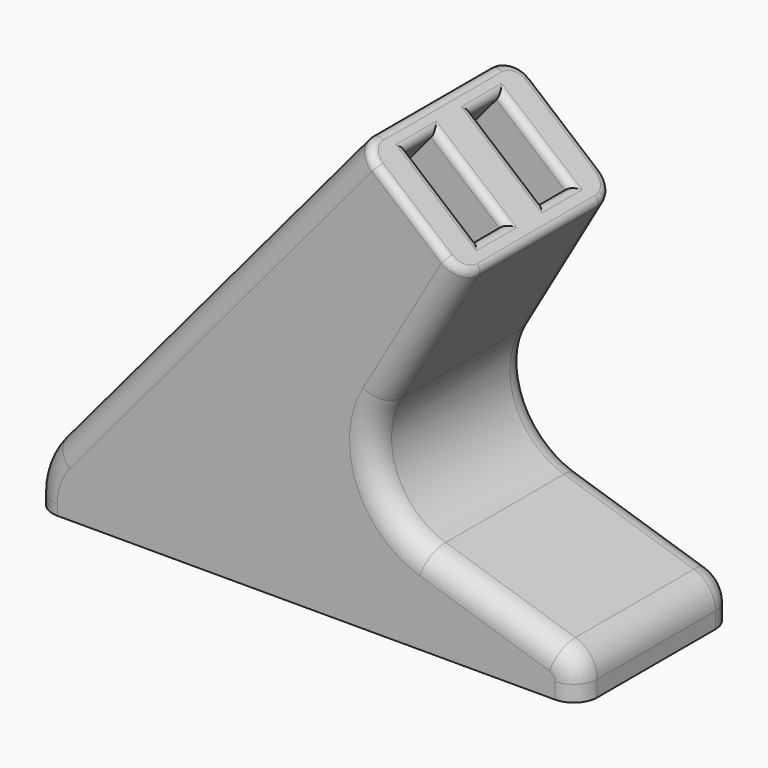
from build123d import *

# Parameters (mm, degrees)
F1_DEPTH      = 12.5
F1_DEPTH_BACK = 12.5
F4_DEPTH      = 4.5
F5_R          = 10
F6_R          = 4
F7_R          = 3
F8_R          = 1


# Not quite as in the source:
# - a pattern or mirror of a feature is missing from the dataset's text; its kind, count and spacing are read off the source's solid


with BuildPart() as f1:
    # F0 (on Front) → F1 (new body, two sides)
    with BuildSketch(Plane.XZ) as f1_sk:
        Polygon((0, 5), (0, 0), (70, 0), (70, 5), (38.7070253131, 15), (55.1869723842, 43.5441056332), (41.7811946296, 54.7928888027), align=None)
    extrude(amount=F1_DEPTH)
    extrude(f1_sk.sketch, amount=-F1_DEPTH_BACK)

    # F3 (on offset) → F4 (cut)
    with BuildSketch(Plane.XZ.offset(3)):
        with BuildLine():
            Line((52.8888390549, 45.4724684623), (44.079327959, 52.8645259737))
            Line((44.079327959, 52.8645259737), (8.0516093002, 9.9283628291))
            ThreePointArc((8.0516093002, 9.9283628291), (7.6308192684, 6.7321452148), (10.3497426295, 5))
            Line((10.3497426295, 5), (11.933790823, 5))
            ThreePointArc((11.933790823, 5), (18.2730647491, 6.4053831945), (23.4244574698, 10.3581858547))
            Line((23.4244574698, 10.3581858547), (52.8888390549, 45.4724684623))
        make_face()
    f4 = extrude(amount=F4_DEPTH, mode=Mode.SUBTRACT)

    # F4_copies: F4 across plane
    add(f4.mirror(Plane.ZX), mode=Mode.SUBTRACT)

    # F5
    f5_edges = [f1.edges().sort_by_distance(p)[0] for p in [
        (38.707025, 0, 15),
        (0, 0, 5),
    ]]
    fillet(f5_edges, radius=F5_R)

    # F6
    f6_edges = [f1.edges().sort_by_distance(p)[0] for p in [
        (70, 0, 5),
    ]]
    fillet(f6_edges, radius=F6_R)

    # F7
    f7_edges = [f1.edges().sort_by_distance(p)[0] for p in [
        (22.060375, -12.5, 31.290531),
        (50.049611, -12.5, 34.645935),
        (50.049611, 12.5, 34.645935),
        (22.060375, 12.5, 31.290531),
        (70, -12.5, 1.039484),
        (69.230351, -12.5, 4.437958),
        (58.873064, -12.5, 8.55573),
        (0, -12.5, 0.680149),
        (44.245427, -12.5, 17.141433),
        (0.603074, -12.5, 4.780499),
        (70, 12.5, 1.039484),
        (69.230351, 12.5, 4.437958),
        (58.873064, 12.5, 8.55573),
        (0, 12.5, 0.680149),
        (44.245427, 12.5, 17.141433),
        (0.603074, 12.5, 4.780499),
    ]]
    fillet(f7_edges, radius=F7_R)

    # F8
    f8_edges = [f1.edges().sort_by_distance(p)[0] for p in [
        (55.186972, 0, 43.544106),
        (54.497154, -11.629423, 44.122932),
        (54.497154, 11.629423, 44.122932),
        (48.466357, -12.5, 49.183371),
        (48.466357, 12.5, 49.183371),
        (42.454302, -11.62132, 54.228084),
        (42.454302, 11.62132, 54.228084),
        (41.781195, 0, 54.792889),
        (52.888839, -5.25, 45.472468),
        (48.484084, -3, 49.168497),
        (48.484084, -7.5, 49.168497),
        (44.079328, -5.25, 52.864526),
        (48.484084, 3, 49.168497),
        (44.079328, 5.25, 52.864526),
        (48.484084, 7.5, 49.168497),
        (52.888839, 5.25, 45.472468),
    ]]
    fillet(f8_edges, radius=F8_R)


solid = f1.part
